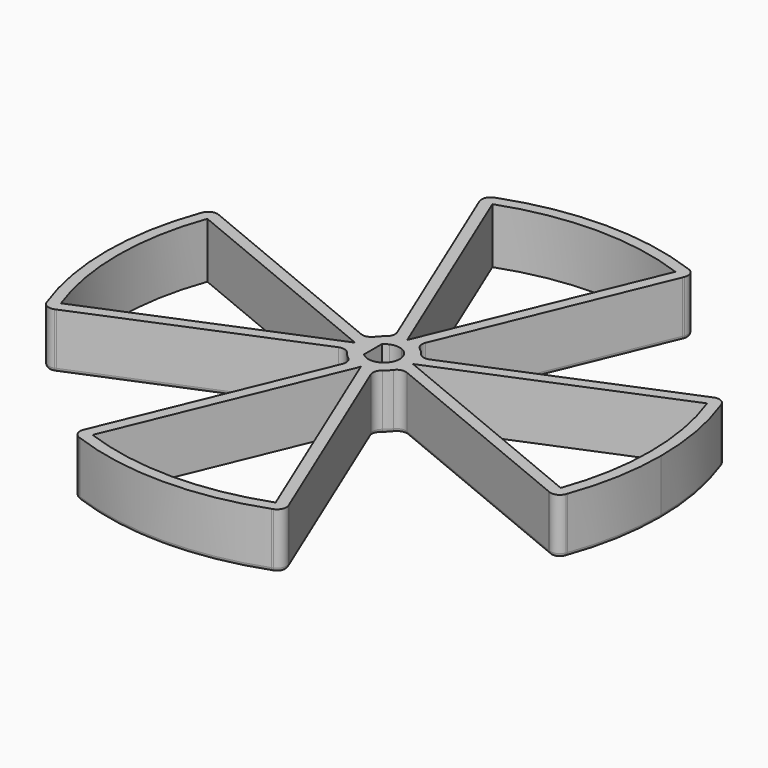
from build123d import *

# Parameters (mm, degrees)
F1_DEPTH = 6
F2_R     = 1
F3_R     = 0.4


# Not quite as in the source:
# - ends of sketch curves that miss each other by under 0.0002 mm in the source are joined


with BuildPart() as f1:
    # F0 (on Top) → F1 (new body)
    with BuildSketch(Plane.XY):
        with BuildLine():
            Line((-11.480502971, 27.7163859753), (-11.0212827483, 26.6077302858))
            ThreePointArc((-11.0212827483, 26.6077302858), (-10.4644415703, 26.8316128289), (-9.9030560674, 27.0438433826))
            Line((-9.9030560674, 27.0438433826), (-10.3626594529, 28.1534241091))
            ThreePointArc((-10.3626594529, 28.1534241091), (-10.9237670586, 27.9404959378), (-11.480502971, 27.7163859753))
        make_face()
        with BuildLine():
            Line((-11.0212827483, 26.6077302858), (-1.2000001632, 2.8970566689))
            ThreePointArc((-1.2000001632, 2.8970566689), (-0.6117547781, 3.0754989557), (0, 3.1357515423))
            Line((0, 3.1357515423), (-9.9030560674, 27.0438433826))
            ThreePointArc((-9.9030560674, 27.0438433826), (-10.4644415703, 26.8316128289), (-11.0212827483, 26.6077302858))
        make_face()
        with BuildLine():
            ThreePointArc((9.9030560674, 27.0438433826), (10.4644415703, 26.8316128289), (11.0212827483, 26.6077302858))
            Line((11.0212827483, 26.6077302858), (11.480502971, 27.7163859753))
            ThreePointArc((11.480502971, 27.7163859753), (10.9237670586, 27.9404959378), (10.3626594529, 28.1534241091))
            Line((10.3626594529, 28.1534241091), (9.9030560674, 27.0438433826))
        make_face()
        with BuildLine():
            ThreePointArc((0, 3.1357515423), (0.6117547781, 3.0754989557), (1.2000001632, 2.8970566689))
            Line((1.2000001632, 2.8970566689), (11.0212827483, 26.6077302858))
            ThreePointArc((11.0212827483, 26.6077302858), (10.4644415703, 26.8316128289), (9.9030560674, 27.0438433826))
            Line((9.9030560674, 27.0438433826), (0, 3.1357515423))
        make_face()
        with BuildLine():
            Line((-1.2000001632, 2.8970566689), (-0.650561835, 1.5705952053))
            ThreePointArc((-0.650561835, 1.5705952053), (0, 1.7), (0.650561835, 1.5705952053))
            Line((0.650561835, 1.5705952053), (1.2000001632, 2.8970566689))
            ThreePointArc((1.2000001632, 2.8970566689), (0.6117547781, 3.0754989557), (0, 3.1357515423))
            ThreePointArc((0, 3.1357515423), (-0.6117547781, 3.0754989557), (-1.2000001632, 2.8970566689))
        make_face()
        with BuildLine():
            Line((-2.8970566689, 1.2000001632), (-1.2, 0.4970562748))
            Line((-1.2, 0.4970562748), (-1.2, 1.2041594579))
            ThreePointArc((-1.2, 1.2041594579), (-0.943246291, 1.4143148286), (-0.650561835, 1.5705952053))
            Line((-0.650561835, 1.5705952053), (-1.2000001632, 2.8970566689))
            ThreePointArc((-1.2000001632, 2.8970566689), (-2.2173111797, 2.2173111797), (-2.8970566689, 1.2000001632))
        make_face()
        with BuildLine():
            Line((-2.8970566689, -1.2000001632), (-1.2, -0.4970562748))
            Line((-1.2, -0.4970562748), (-1.2, 0.4970562748))
            Line((-1.2, 0.4970562748), (-2.8970566689, 1.2000001632))
            ThreePointArc((-2.8970566689, 1.2000001632), (-3.0754989557, 0.6117547781), (-3.1357515423, 0))
            ThreePointArc((-3.1357515423, 0), (-3.0754989557, -0.6117547781), (-2.8970566689, -1.2000001632))
        make_face()
        with BuildLine():
            ThreePointArc((-3.1357515423, 0), (-3.0754989557, 0.6117547781), (-2.8970566689, 1.2000001632))
            Line((-2.8970566689, 1.2000001632), (-26.6077302858, 11.0212827483))
            ThreePointArc((-26.6077302858, 11.0212827483), (-26.8316128289, 10.4644415703), (-27.0438433826, 9.9030560674))
            Line((-27.0438433826, 9.9030560674), (-3.1357515423, 0))
        make_face()
        with BuildLine():
            ThreePointArc((-27.0438433826, 9.9030560674), (-26.8316128289, 10.4644415703), (-26.6077302858, 11.0212827483))
            Line((-26.6077302858, 11.0212827483), (-27.7163859753, 11.480502971))
            ThreePointArc((-27.7163859753, 11.480502971), (-27.9404959378, 10.9237670586), (-28.1534241091, 10.3626594529))
            Line((-28.1534241091, 10.3626594529), (-27.0438433826, 9.9030560674))
        make_face()
        with BuildLine():
            Line((-27.7163859753, -11.480502971), (-26.6077302858, -11.0212827483))
            ThreePointArc((-26.6077302858, -11.0212827483), (-26.8316128289, -10.4644415703), (-27.0438433826, -9.9030560674))
            Line((-27.0438433826, -9.9030560674), (-28.1534241091, -10.3626594529))
            ThreePointArc((-28.1534241091, -10.3626594529), (-27.9404959378, -10.9237670586), (-27.7163859753, -11.480502971))
        make_face()
        with BuildLine():
            ThreePointArc((0, -3.1357515423), (-0.6117547781, -3.0754989557), (-1.2000001632, -2.8970566689))
            Line((-1.2000001632, -2.8970566689), (-11.0212827483, -26.6077302858))
            ThreePointArc((-11.0212827483, -26.6077302858), (-10.4644415703, -26.8316128289), (-9.9030560674, -27.0438433826))
            Line((-9.9030560674, -27.0438433826), (0, -3.1357515423))
        make_face()
        with BuildLine():
            ThreePointArc((-9.9030560674, -27.0438433826), (-10.4644415703, -26.8316128289), (-11.0212827483, -26.6077302858))
            Line((-11.0212827483, -26.6077302858), (-11.480502971, -27.7163859753))
            ThreePointArc((-11.480502971, -27.7163859753), (-10.9237670586, -27.9404959378), (-10.3626594529, -28.1534241091))
            Line((-10.3626594529, -28.1534241091), (-9.9030560674, -27.0438433826))
        make_face()
        with BuildLine():
            Line((11.480502971, -27.7163859753), (11.0212827483, -26.6077302858))
            ThreePointArc((11.0212827483, -26.6077302858), (10.4644415703, -26.8316128289), (9.9030560674, -27.0438433826))
            Line((9.9030560674, -27.0438433826), (10.3626594529, -28.1534241091))
            ThreePointArc((10.3626594529, -28.1534241091), (10.9237670586, -27.9404959378), (11.480502971, -27.7163859753))
        make_face()
        with BuildLine():
            ThreePointArc((0.650561835, -1.5705952053), (0, -1.7), (-0.650561835, -1.5705952053))
            Line((-0.650561835, -1.5705952053), (-1.2000001632, -2.8970566689))
            ThreePointArc((-1.2000001632, -2.8970566689), (-0.6117547781, -3.0754989557), (0, -3.1357515423))
            ThreePointArc((0, -3.1357515423), (0.6117547781, -3.0754989557), (1.2000001632, -2.8970566689))
            Line((1.2000001632, -2.8970566689), (0.650561835, -1.5705952053))
        make_face()
        with BuildLine():
            ThreePointArc((1.5705952053, -0.650561835), (1.202081528, -1.202081528), (0.650561835, -1.5705952053))
            Line((0.650561835, -1.5705952053), (1.2000001632, -2.8970566689))
            ThreePointArc((1.2000001632, -2.8970566689), (2.2173111797, -2.2173111797), (2.8970566689, -1.2000001632))
            Line((2.8970566689, -1.2000001632), (1.5705952053, -0.650561835))
        make_face()
        with BuildLine():
            ThreePointArc((1.5705952053, 0.650561835), (1.7, 0), (1.5705952053, -0.650561835))
            Line((1.5705952053, -0.650561835), (2.8970566689, -1.2000001632))
            ThreePointArc((2.8970566689, -1.2000001632), (3.0754989557, -0.6117547781), (3.1357515423, 0))
            ThreePointArc((3.1357515423, 0), (3.0754989557, 0.6117547781), (2.8970566689, 1.2000001632))
            Line((2.8970566689, 1.2000001632), (1.5705952053, 0.650561835))
        make_face()
        with BuildLine():
            Line((1.2000001632, 2.8970566689), (0.650561835, 1.5705952053))
            ThreePointArc((0.650561835, 1.5705952053), (1.202081528, 1.202081528), (1.5705952053, 0.650561835))
            Line((1.5705952053, 0.650561835), (2.8970566689, 1.2000001632))
            ThreePointArc((2.8970566689, 1.2000001632), (2.2173111797, 2.2173111797), (1.2000001632, 2.8970566689))
        make_face()
        with BuildLine():
            Line((26.6077302858, 11.0212827483), (2.8970566689, 1.2000001632))
            ThreePointArc((2.8970566689, 1.2000001632), (3.0754989557, 0.6117547781), (3.1357515423, 0))
            Line((3.1357515423, 0), (27.0438433826, 9.9030560674))
            ThreePointArc((27.0438433826, 9.9030560674), (26.8316128289, 10.4644415703), (26.6077302858, 11.0212827483))
        make_face()
        with BuildLine():
            Line((27.7163859753, 11.480502971), (26.6077302858, 11.0212827483))
            ThreePointArc((26.6077302858, 11.0212827483), (26.8316128289, 10.4644415703), (27.0438433826, 9.9030560674))
            Line((27.0438433826, 9.9030560674), (28.1534241091, 10.3626594529))
            ThreePointArc((28.1534241091, 10.3626594529), (27.9404959378, 10.9237670586), (27.7163859753, 11.480502971))
        make_face()
        with BuildLine():
            ThreePointArc((3.1357515423, 0), (3.0754989557, -0.6117547781), (2.8970566689, -1.2000001632))
            Line((2.8970566689, -1.2000001632), (26.6077302858, -11.0212827483))
            ThreePointArc((26.6077302858, -11.0212827483), (26.8316128289, -10.4644415703), (27.0438433826, -9.9030560674))
            Line((27.0438433826, -9.9030560674), (3.1357515423, 0))
        make_face()
        with BuildLine():
            ThreePointArc((27.0438433826, -9.9030560674), (26.8316128289, -10.4644415703), (26.6077302858, -11.0212827483))
            Line((26.6077302858, -11.0212827483), (27.7163859753, -11.480502971))
            ThreePointArc((27.7163859753, -11.480502971), (27.9404959378, -10.9237670586), (28.1534241091, -10.3626594529))
            Line((28.1534241091, -10.3626594529), (27.0438433826, -9.9030560674))
        make_face()
        with BuildLine():
            ThreePointArc((-0.650561835, -1.5705952053), (-0.943246291, -1.4143148286), (-1.2, -1.2041594579))
            Line((-1.2, -1.2041594579), (-1.2, -0.4970562748))
            Line((-1.2, -0.4970562748), (-2.8970566689, -1.2000001632))
            ThreePointArc((-2.8970566689, -1.2000001632), (-2.2173111797, -2.2173111797), (-1.2000001632, -2.8970566689))
            Line((-1.2000001632, -2.8970566689), (-0.650561835, -1.5705952053))
        make_face()
        with BuildLine():
            Line((11.0212827483, -26.6077302858), (1.2000001632, -2.8970566689))
            ThreePointArc((1.2000001632, -2.8970566689), (0.6117547781, -3.0754989557), (0, -3.1357515423))
            Line((0, -3.1357515423), (9.9030560674, -27.0438433826))
            ThreePointArc((9.9030560674, -27.0438433826), (10.4644415703, -26.8316128289), (11.0212827483, -26.6077302858))
        make_face()
        with BuildLine():
            Line((-26.6077302858, -11.0212827483), (-2.8970566689, -1.2000001632))
            ThreePointArc((-2.8970566689, -1.2000001632), (-3.0754989557, -0.6117547781), (-3.1357515423, 0))
            Line((-3.1357515423, 0), (-27.0438433826, -9.9030560674))
            ThreePointArc((-27.0438433826, -9.9030560674), (-26.8316128289, -10.4644415703), (-26.6077302858, -11.0212827483))
        make_face()
        with BuildLine():
            Line((-10.3626594529, 28.1534241091), (-9.9030560674, 27.0438433826))
            ThreePointArc((-9.9030560674, 27.0438433826), (0, 28.7999997288), (9.9030560674, 27.0438433826))
            Line((9.9030560674, 27.0438433826), (10.3626594529, 28.1534241091))
            ThreePointArc((10.3626594529, 28.1534241091), (0, 30), (-10.3626594529, 28.1534241091))
        make_face()
        with BuildLine():
            ThreePointArc((-27.0438433826, -9.9030560674), (-28.7999997288, 0), (-27.0438433826, 9.9030560674))
            Line((-27.0438433826, 9.9030560674), (-28.1534241091, 10.3626594529))
            ThreePointArc((-28.1534241091, 10.3626594529), (-30, 0), (-28.1534241091, -10.3626594529))
            Line((-28.1534241091, -10.3626594529), (-27.0438433826, -9.9030560674))
        make_face()
        with BuildLine():
            Line((10.3626594529, -28.1534241091), (9.9030560674, -27.0438433826))
            ThreePointArc((9.9030560674, -27.0438433826), (0, -28.7999997288), (-9.9030560674, -27.0438433826))
            Line((-9.9030560674, -27.0438433826), (-10.3626594529, -28.1534241091))
            ThreePointArc((-10.3626594529, -28.1534241091), (0, -30), (10.3626594529, -28.1534241091))
        make_face()
        with BuildLine():
            ThreePointArc((28.7999997288, 0), (28.3575621878, -5.0287822727), (27.0438433826, -9.9030560674))
            Line((27.0438433826, -9.9030560674), (28.1534241091, -10.3626594529))
            ThreePointArc((28.1534241091, -10.3626594529), (29.534748376, -5.2629495878), (30, 0))
            ThreePointArc((30, 0), (29.534748376, 5.2629495878), (28.1534241091, 10.3626594529))
            Line((28.1534241091, 10.3626594529), (27.0438433826, 9.9030560674))
            ThreePointArc((27.0438433826, 9.9030560674), (28.3575621878, 5.0287822727), (28.7999997288, 0))
        make_face()
    extrude(amount=F1_DEPTH)

    # F2
    f2_edges = [f1.edges().sort_by_distance(p)[0] for p in [
        (-11.480503, 27.716386, 3),
        (11.480503, 27.716386, 3),
        (-27.716386, 11.480503, 3),
        (-1.2, 2.897057, 3),
        (-2.897057, 1.2, 3),
        (-27.716386, -11.480503, 3),
        (-11.480503, -27.716386, 3),
        (27.716386, 11.480503, 3),
        (-2.897057, -1.2, 3),
        (-1.2, -2.897057, 3),
        (1.2, -2.897057, 3),
        (2.897057, -1.2, 3),
        (11.480503, -27.716386, 3),
        (27.716386, -11.480503, 3),
        (1.2, 2.897057, 3),
        (2.897057, 1.2, 3),
    ]]
    fillet(f2_edges, radius=F2_R)

    # F3
    f3_edges = [f1.edges().sort_by_distance(p)[0] for p in [
        (-1.2, 0, 0),
        (1.7, 0, 0),
        (-3.057575, -1.495988, 0),
    ]]
    fillet(f3_edges, radius=F3_R)


solid = f1.part
